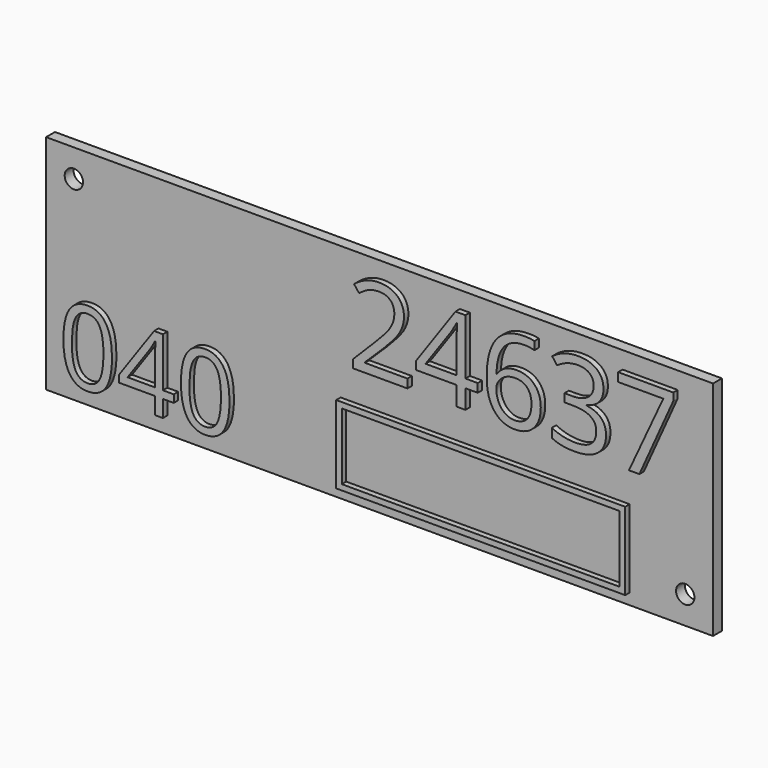
from build123d import *

# Parameters (mm, degrees)
F0_W         = 120
F0_H         = 40
F1_DEPTH     = 2
F3_D         = 3.3
F4_TEXT_SIZE = 20.8865923307
F5_DEPTH     = 1
F6_TEXT_SIZE = 18.4937691891
F7_DEPTH     = 1
F8_W         = 52
F8_H         = 14
F8_W_2       = 49.99999962
F8_H_2       = 11.99999962
F9_DEPTH     = 1


# Not quite as in the source:
# - Text() gives the source's letters only with a copy of the font that has no kerning and outlines rounded to 1/6400 em; it was checked with that copy


with BuildPart() as f1:
    # F0 (on Front) → F1 (new body)
    with BuildSketch(Plane.XZ):
        Rectangle(F0_W, F0_H)
    extrude(amount=F1_DEPTH)

    # F3 (through all)
    with Locations(Plane.XZ.offset(2)):
        with Locations((-55, 15), (55, -15)):
            Hole(F3_D / 2)

    # F4 (on face) → F5 (join)
    with BuildSketch(Plane.XZ.offset(2)):
        with Locations((-5, 2)):
            Text('24637', F4_TEXT_SIZE, font='Open Sans', text_align=(TextAlign.LEFT, TextAlign.BOTTOM))
    extrude(amount=F5_DEPTH)

    # F6 (on face) → F7 (join)
    with BuildSketch(Plane.XZ.offset(2)):
        with Locations((-57, -17)):
            Text('040', F6_TEXT_SIZE, font='Open Sans', text_align=(TextAlign.LEFT, TextAlign.BOTTOM))
    extrude(amount=F7_DEPTH)

    # F8 (on face) → F9 (join)
    with BuildSketch(Plane.XZ.offset(2)):
        with Locations((19, -11)):
            Rectangle(F8_W, F8_H)
        with Locations((19, -11)):
            Rectangle(F8_W_2, F8_H_2, mode=Mode.SUBTRACT)
    extrude(amount=F9_DEPTH)


solid = f1.part
